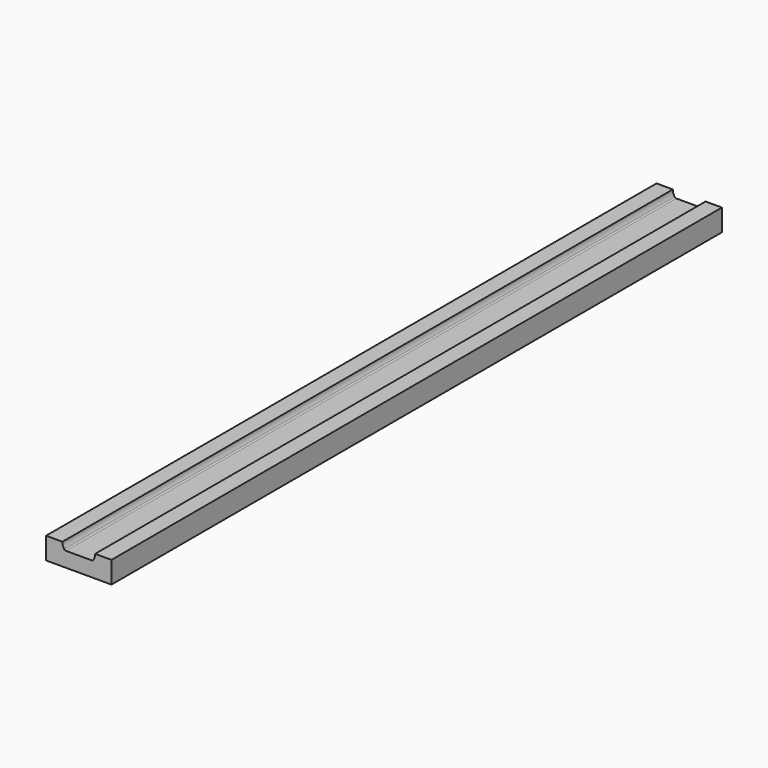
from build123d import *

# Parameters (mm, degrees)
F1_DEPTH = 1400


# Not quite as in the source:
# - ends of sketch curves that miss each other by under 0.0002 mm in the source are joined


with BuildPart() as f1:
    # F0 (on Front) → F1 (new body)
    with BuildSketch(Plane.XZ):
        with BuildLine():
            ThreePointArc((-102.8194582262, -1.753334156), (-102.8759917705, -1.6691495307), (-102.9300627594, -1.5833624634))
            ThreePointArc((-102.9300627594, -1.5833624634), (-105.3062912412, 3.621474375), (-106.1115923498, 9.2861260008))
            Line((-106.1115923498, 9.2861260008), (-136.111652, 9.288465))
            Line((-136.111652, 9.288465), (-136.111652, -30.711535))
            Line((-136.111652, -30.711535), (-16.111652, -30.711535))
            Line((-16.111652, -30.711535), (-16.111652, 9.288465))
            Line((-16.111652, 9.288465), (-46.111705, 9.288465))
            ThreePointArc((-46.111705, 9.288465), (-46.9260256459, 3.5907327912), (-49.3292641557, -1.6391538962))
            ThreePointArc((-49.3292641557, -1.6391538962), (-49.348739835, -1.6694199812), (-49.3685261016, -1.6994839384))
            ThreePointArc((-49.3685261016, -1.6994839384), (-50.6166534947, -2.8386108222), (-52.2530199988, -3.2601991421))
            Line((-52.2530199988, -3.2601991421), (-52.3114330011, -3.260199))
            Line((-52.3114330011, -3.260199), (-99.942409, -3.260199))
            ThreePointArc((-99.942409, -3.260199), (-101.566297382, -2.8606806598), (-102.8194582262, -1.753334156))
        make_face()
    extrude(amount=F1_DEPTH)


solid = f1.part
